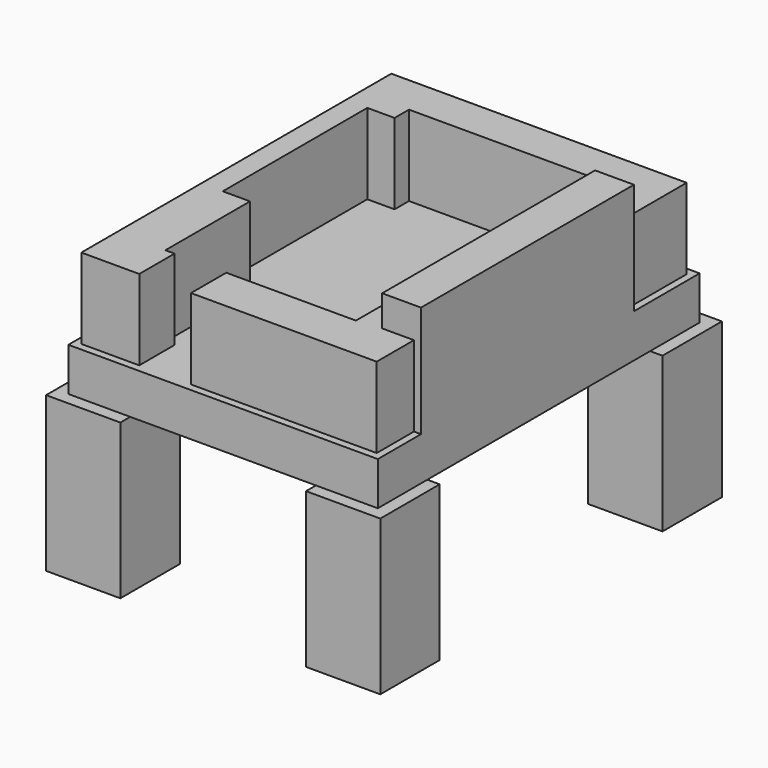
from build123d import *

# Parameters (mm, degrees)
F0_R         = 0.83
F1_DEPTH     = 7
F3_DEPTH     = 20
F0_W         = 6.2750220299
F0_H         = 43
F4_DEPTH     = 25
F5_T         = 2.5
F5_T3_DEPTH  = 6.139113307
F5_T5_DEPTH  = 17.0775900483
F5_T7_DEPTH  = 52.7217752486
F5_T9_DEPTH  = 67.6008063555
F5_T11_DEPTH = 14.360413067
F5_T13_DEPTH = 12.124489639
F5_T15_DEPTH = 6.4792522416
F5_T17_DEPTH = 22.0955071226
F5_T19_DEPTH = 9.4071413577
F5_T21_DEPTH = 34.1892816313
F5_T23_DEPTH = 7.9103027191
F5_T25_DEPTH = 35.7827994693
F5_T27_DEPTH = 54.1950914729
F5_T29_DEPTH = 25.949822152
F5_T31_DEPTH = 35.0076371059
F5_T33_DEPTH = 12.5232163072
F5_T35_DEPTH = 10.1359087229
F5_T37_DEPTH = 18
F6_W         = 12
F6_H         = 12
F7_DEPTH     = 25


# Not quite as in the source:
# - a shell that OpenCascade refuses in one call is made with other operations: the cavity is built on its own and cut out


with BuildPart() as f1:
    # F0 (on Top) → F1 (new body)
    with BuildSketch(Plane.XY):
        Polygon((25, 32.5), (-25, 32.5), (-25, -32.5), (25, -32.5), (25, -23.7771868706), (18.7249779701, -23.7771868706), (18.7249779701, 19.2228131294), (25, 19.2228131294), align=None)
        with Locations((0.16, -3)):
            Circle(F0_R, mode=Mode.SUBTRACT)
        with Locations((2.7, -3)):
            Circle(F0_R, mode=Mode.SUBTRACT)
        with Locations((0.16, -0.46)):
            Circle(F0_R, mode=Mode.SUBTRACT)
        with Locations((2.7, -0.46)):
            Circle(F0_R, mode=Mode.SUBTRACT)
        with Locations((0.16, 2.08)):
            Circle(F0_R, mode=Mode.SUBTRACT)
        with Locations((2.7, 2.08)):
            Circle(F0_R, mode=Mode.SUBTRACT)
    extrude(amount=F1_DEPTH)

    # F2 (on Top) → F3 (join)
    with BuildSketch(Plane.XY):
        Polygon((23.860886693, 31.3004031777), (-23.8608885556, 31.3004031777), (-23.8608885556, -31.3004031777), (-14.5004754886, -31.3004031777), (-14.5004754886, -24.1759135388), (-15.9797277302, -24.1759135388), (-15.9797277302, -7.0804064162), (-20.3868690878, -7.0804064162), (-20.3868690878, 22.1088752151), (-15.9797277302, 22.1088752151), (-15.9797277302, 25.0191779342), (14.8030717392, 25.0191779342), (14.8030717392, -24.1759135388), (-6.1467504129, -24.1759135388), (-6.1467504129, -31.3004031777), (23.860886693, -31.3004031777), align=None)
    extrude(amount=F3_DEPTH)

    # F0 (on Top) → F4 (join)
    with BuildSketch(Plane.XY):
        with Locations((21.8624889851, -2.2771868706)):
            Rectangle(F0_W, F0_H)
    extrude(amount=F4_DEPTH)

    # F5: shell of thickness 2.5, made by hand


with BuildPart() as f5_core1:
    # F5_t2: copy of F1
    add(f1.part)

    # the walls: a layer under each face that stays
    f5_faces = [f5_core1.faces().sort_by_distance(p)[0] for p in [
        (0, 32.5, 3.5),
        (-16.6666666667, 0, 7),
        (1.87, 2.08, 3.5),
        (1.87, -0.46, 3.5),
        (-0.67, 2.08, 3.5),
        (-0.67, -0.46, 3.5),
        (1.87, -3, 3.5),
        (-0.67, -3, 3.5),
        (0, -32.5, 3.5),
        (19.7708149751, -23.7771868706, 22),
        (21.8624889851, -2.2771868706, 25),
        (15.9072574849, -20.8669354518, 20),
        (23.860886693, -27.5387950242, 13.5),
        (8.8570681401, -31.3004031777, 13.5),
        (-6.1467504129, -27.7381583583, 13.5),
        (4.3281606631, -24.1759135388, 13.5),
        (14.8030717392, 0.4216321977, 13.5),
        (-0.5883279955, 25.0191779342, 13.5),
        (-15.9797277302, 23.5640265746, 13.5),
        (-18.183298409, 22.1088752151, 13.5),
        (-20.3868690878, 7.5142343994, 13.5),
        (-18.183298409, -7.0804064162, 13.5),
        (-15.9797277302, -15.6281599775, 13.5),
        (-15.2401016094, -24.1759135388, 13.5),
        (-14.5004754886, -27.7381583583, 13.5),
        (-19.1806820221, -31.3004031777, 13.5),
        (-23.8608885556, 0, 13.5),
        (-9.313e-07, 31.3004031777, 13.5),
        (23.860886693, 25.2616081536, 13.5),
        (23.954162995, 19.2228131294, 22),
        (-16.6666666667, -21.6666666667, 0),
        (-25, 0, 3.5),
        (25, 0, 12.5),
    ]]
    thicken(f5_faces, amount=-F5_T, mode=Mode.SUBTRACT)

    # F5_s4 → F5_t3 (cut)
    with BuildSketch(Plane.YZ.offset(21.360886693)):
        Polygon((19.2478131294, 7.025), (19.2228131294, 4.5), (16.7228131294, 4.5), (16.7228131294, 7), align=None)
        Polygon((-23.8021868706, 7.025), (-23.7771868706, 4.5), (-21.2771868706, 4.5), (-21.2771868706, 7), align=None)
    extrude(amount=F5_T3_DEPTH, mode=Mode.SUBTRACT)

    # F5_s6 → F5_t5 (cut)
    with BuildSketch(Plane.XZ.offset(-33.8004031777)):
        Polygon((23.885886693, 7.025), (23.860886693, 4.5), (21.360886693, 4.5), (21.360886693, 7), align=None)
    extrude(amount=F5_T5_DEPTH, mode=Mode.SUBTRACT)

    # F5_s8 → F5_t7 (cut)
    with BuildSketch(Plane.YZ.offset(-26.3608885556)):
        Polygon((31.3254031777, 7.025), (31.3004031777, 4.5), (28.8004031777, 4.5), (28.8004031777, 7), align=None)
    extrude(amount=F5_T7_DEPTH, mode=Mode.SUBTRACT)

    # F5_s10 → F5_t9 (cut)
    with BuildSketch(Plane.XZ.offset(-33.8004031777)):
        Polygon((-23.8858885556, 7.025), (-23.8608885556, 4.5), (-21.3608885556, 4.5), (-21.3608885556, 7), align=None)
    extrude(amount=F5_T9_DEPTH, mode=Mode.SUBTRACT)

    # F5_s12 → F5_t11 (cut)
    with BuildSketch(Plane.YZ.offset(-26.3608885556)):
        Polygon((-31.3254031777, 7.025), (-31.3004031777, 4.5), (-28.8004031777, 4.5), (-28.8004031777, 7), align=None)
    extrude(amount=F5_T11_DEPTH, mode=Mode.SUBTRACT)

    # F5_s14 → F5_t13 (cut)
    with BuildSketch(Plane.XZ.offset(21.6759135388)):
        Polygon((-14.4754754886, 7.025), (-14.5004754886, 4.5), (-17.0004754886, 4.5), (-17.0004754886, 7), align=None)
        Polygon((-6.1717504129, 7.025), (-6.1467504129, 4.5), (-3.6467504129, 4.5), (-3.6467504129, 7), align=None)
    extrude(amount=F5_T13_DEPTH, mode=Mode.SUBTRACT)

    # F5_s16 → F5_t15 (cut)
    with BuildSketch(Plane.YZ.offset(-18.4797277302)):
        Polygon((-24.1509135388, 7.025), (-24.1759135388, 4.5), (-26.6759135388, 4.5), (-26.6759135388, 7), align=None)
    extrude(amount=F5_T15_DEPTH, mode=Mode.SUBTRACT)

    # F5_s18 → F5_t17 (cut)
    with BuildSketch(Plane.XZ.offset(4.5804064162)):
        Polygon((-15.9547277302, 7.025), (-15.9797277302, 4.5), (-18.4797277302, 4.5), (-18.4797277302, 7), align=None)
    extrude(amount=F5_T17_DEPTH, mode=Mode.SUBTRACT)

    # F5_s20 → F5_t19 (cut)
    with BuildSketch(Plane.YZ.offset(-22.8868690878)):
        Polygon((-7.0554064162, 7.025), (-7.0804064162, 4.5), (-9.5804064162, 4.5), (-9.5804064162, 7), align=None)
        Polygon((22.0838752151, 7.025), (22.1088752151, 4.5), (24.6088752151, 4.5), (24.6088752151, 7), align=None)
    extrude(amount=F5_T19_DEPTH, mode=Mode.SUBTRACT)

    # F5_s22 → F5_t21 (cut)
    with BuildSketch(Plane.XZ.offset(-24.6088752151)):
        Polygon((-20.3618690878, 7.025), (-20.3868690878, 4.5), (-22.8868690878, 4.5), (-22.8868690878, 7), align=None)
    extrude(amount=F5_T21_DEPTH, mode=Mode.SUBTRACT)

    # F5_s24 → F5_t23 (cut)
    with BuildSketch(Plane.XZ.offset(-27.5191779342)):
        Polygon((-15.9547277302, 7.025), (-15.9797277302, 4.5), (-18.4797277302, 4.5), (-18.4797277302, 7), align=None)
    extrude(amount=F5_T23_DEPTH, mode=Mode.SUBTRACT)

    # F5_s26 → F5_t25 (cut)
    with BuildSketch(Plane.YZ.offset(-18.4797277302)):
        Polygon((24.9941779342, 7.025), (25.0191779342, 4.5), (27.5191779342, 4.5), (27.5191779342, 7), align=None)
    extrude(amount=F5_T25_DEPTH, mode=Mode.SUBTRACT)

    # F5_s28 → F5_t27 (cut)
    with BuildSketch(Plane.XZ.offset(-27.5191779342)):
        Polygon((14.7780717392, 7.025), (14.8030717392, 4.5), (17.3030717392, 4.5), (17.3030717392, 7), align=None)
    extrude(amount=F5_T27_DEPTH, mode=Mode.SUBTRACT)

    # F5_s30 → F5_t29 (cut)
    with BuildSketch(Plane.YZ.offset(-8.6467504129)):
        Polygon((-24.1509135388, 7.025), (-24.1759135388, 4.5), (-26.6759135388, 4.5), (-26.6759135388, 7), align=None)
    extrude(amount=F5_T29_DEPTH, mode=Mode.SUBTRACT)

    # F5_s32 → F5_t31 (cut)
    with BuildSketch(Plane.YZ.offset(-8.6467504129)):
        Polygon((-31.3254031777, 7.025), (-31.3004031777, 4.5), (-28.8004031777, 4.5), (-28.8004031777, 7), align=None)
    extrude(amount=F5_T31_DEPTH, mode=Mode.SUBTRACT)

    # F5_s34 → F5_t33 (cut)
    with BuildSketch(Plane.XZ.offset(21.2771868706)):
        Polygon((23.885886693, 7.025), (23.860886693, 4.5), (21.360886693, 4.5), (21.360886693, 7), align=None)
    extrude(amount=F5_T33_DEPTH, mode=Mode.SUBTRACT)

    # F5_s36 → F5_t35 (cut)
    with BuildSketch(Plane.YZ.offset(16.2249779701)):
        Polygon((-23.8021868706, 20.025), (-21.2771868706, 20), (-21.2771868706, 17.5), (-23.7771868706, 17.5), align=None)
        Polygon((19.2478131294, 20.025), (19.2228131294, 17.5), (16.7228131294, 17.5), (16.7228131294, 20), align=None)
    extrude(amount=F5_T35_DEPTH, mode=Mode.SUBTRACT)

    # F5_s38 → F5_t37 (cut)
    with BuildSketch(Plane.XY.offset(4.5)):
        Polygon((23.885886693, -23.8021868706), (23.860886693, -21.2771868706), (21.360886693, -21.2771868706), (21.360886693, -23.7771868706), align=None)
        Polygon((14.7780717392, -24.1509135388), (14.8030717392, -26.6759135388), (17.3030717392, -26.6759135388), (17.3030717392, -24.1759135388), align=None)
        Polygon((14.7780717392, 24.9941779342), (17.3030717392, 25.0191779342), (17.3030717392, 27.5191779342), (14.8030717392, 27.5191779342), align=None)
        Polygon((-15.9547277302, 24.9941779342), (-15.9797277302, 27.5191779342), (-18.4797277302, 27.5191779342), (-18.4797277302, 25.0191779342), align=None)
        Polygon((-20.3618690878, 22.0838752151), (-20.3868690878, 24.6088752151), (-22.8868690878, 24.6088752151), (-22.8868690878, 22.1088752151), align=None)
        Polygon((-20.3618690878, -7.0554064162), (-22.8868690878, -7.0804064162), (-22.8868690878, -9.5804064162), (-20.3868690878, -9.5804064162), align=None)
        Polygon((-15.9547277302, -24.1509135388), (-18.4797277302, -24.1759135388), (-18.4797277302, -26.6759135388), (-15.9797277302, -26.6759135388), align=None)
        Polygon((23.885886693, 19.2478131294), (21.360886693, 19.2228131294), (21.360886693, 16.7228131294), (23.860886693, 16.7228131294), align=None)
    extrude(amount=F5_T37_DEPTH, mode=Mode.SUBTRACT)


with BuildPart() as f1_1:
    add(f1.part)

    # what is left inside the walls is the cavity
    f5_cavity = [f5_core1.part.solids().sort_by_distance(p)[0] for p in [
        (0, -10, 2.525),
    ]]
    add(f5_cavity, mode=Mode.SUBTRACT)

    # F6 (on Top) → F7 (join)
    with BuildSketch(Plane.XY):
        with Locations((-21, 28.5)):
            Rectangle(F6_W, F6_H)
        with Locations((-21, -28.5)):
            Rectangle(F6_W, F6_H)
        with Locations((21, -28.5)):
            Rectangle(F6_W, F6_H)
        with Locations((21, 28.5)):
            Rectangle(F6_W, F6_H)
    extrude(amount=-F7_DEPTH)


solid = f1_1.part
